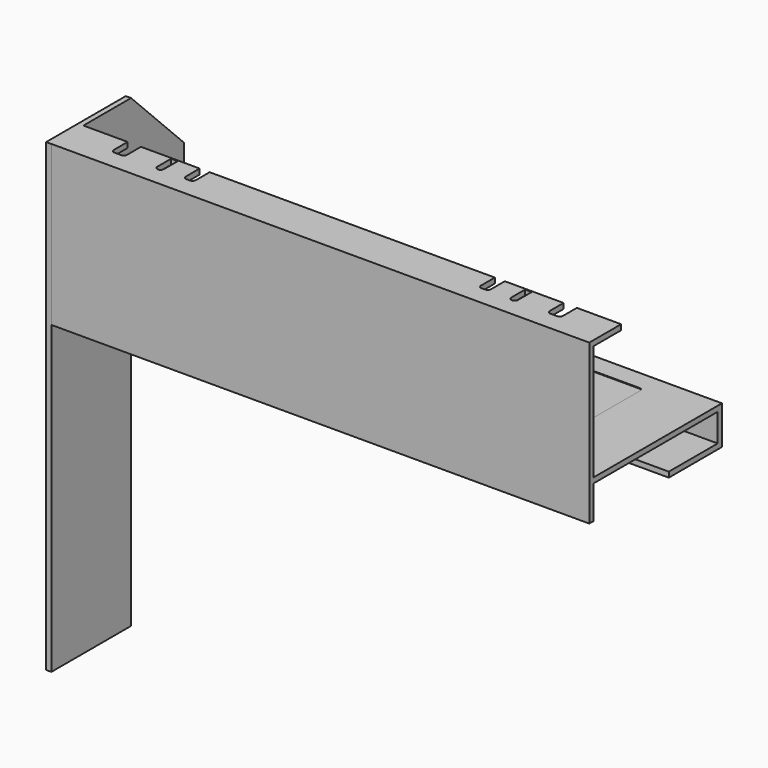
from build123d import *

# Parameters (mm, degrees)
F1_DEPTH = 16
F3_W     = 1620
F3_H     = 484
F4_DEPTH = 16
F5_DEPTH = 14
F6_W     = 184
F6_H     = 16
F6_W_2   = 16
F6_H_2   = 464
F7_DEPTH = 1620
F9_DEPTH = 25


# Not quite as in the source:
# - a feature names something its author has since deleted; it is built from what else it names


with BuildPart() as f1:
    # F0 (on Right) → F1 (new body)
    with BuildSketch(Plane.YZ):
        Polygon((0, 480), (-300, 480), (-300, -920), (0, -920), (0, 0), (200, 0), (200, 280), align=None)
    extrude(amount=-F1_DEPTH)

    # F3 (on offset) → F4 (join)
    with BuildSketch(Plane.XY.offset(100)):
        with Locations((810, -42)):
            Rectangle(F3_W, F3_H)
        with BuildLine():
            Line((200, 140), (680, 140))
            ThreePointArc((680, 140), (687.0710678119, 137.0710678119), (690, 130))
            Line((690, 130), (690, -150))
            ThreePointArc((690, -150), (687.0710678119, -157.0710678119), (680, -160))
            Line((680, -160), (200, -160))
            ThreePointArc((200, -160), (192.9289321881, -157.0710678119), (190, -150))
            Line((190, -150), (190, 130))
            ThreePointArc((190, 130), (192.9289321881, 137.0710678119), (200, 140))
        make_face(mode=Mode.SUBTRACT)
        with BuildLine():
            Line((940, 140), (1420, 140))
            ThreePointArc((1420, 140), (1427.0710678119, 137.0710678119), (1430, 130))
            Line((1430, 130), (1430, -150))
            ThreePointArc((1430, -150), (1427.0710678119, -157.0710678119), (1420, -160))
            Line((1420, -160), (940, -160))
            ThreePointArc((940, -160), (932.9289321881, -157.0710678119), (930, -150))
            Line((930, -150), (930, 130))
            ThreePointArc((930, 130), (932.9289321881, 137.0710678119), (940, 140))
        make_face(mode=Mode.SUBTRACT)
    extrude(amount=F4_DEPTH)

    # F3 (on offset) → F5 (join)
    with BuildSketch(Plane.XY.offset(100)):
        with BuildLine():
            ThreePointArc((690, 130), (687.0710678119, 137.0710678119), (680, 140))
            Line((680, 140), (200, 140))
            ThreePointArc((200, 140), (192.9289321881, 137.0710678119), (190, 130))
            Line((190, 130), (190, -150))
            ThreePointArc((190, -150), (192.9289321881, -157.0710678119), (200, -160))
            Line((200, -160), (680, -160))
            ThreePointArc((680, -160), (687.0710678119, -157.0710678119), (690, -150))
            Line((690, -150), (690, 130))
        make_face()
        with BuildLine():
            ThreePointArc((682, -150), (681.4142135624, -151.4142135624), (680, -152))
            Line((680, -152), (200, -152))
            ThreePointArc((200, -152), (198.5857864376, -151.4142135624), (198, -150))
            Line((198, -150), (198, 130))
            ThreePointArc((198, 130), (198.5857864376, 131.4142135624), (200, 132))
            Line((200, 132), (680, 132))
            ThreePointArc((680, 132), (681.4142135624, 131.4142135624), (682, 130))
            Line((682, 130), (682, -150))
        make_face(mode=Mode.SUBTRACT)
        with BuildLine():
            ThreePointArc((1430, 130), (1427.0710678119, 137.0710678119), (1420, 140))
            Line((1420, 140), (940, 140))
            ThreePointArc((940, 140), (932.9289321881, 137.0710678119), (930, 130))
            Line((930, 130), (930, -150))
            ThreePointArc((930, -150), (932.9289321881, -157.0710678119), (940, -160))
            Line((940, -160), (1420, -160))
            ThreePointArc((1420, -160), (1427.0710678119, -157.0710678119), (1430, -150))
            Line((1430, -150), (1430, 130))
        make_face()
    extrude(amount=F5_DEPTH)

    # F6 (on face) → F7 (join)
    with BuildSketch(Plane.YZ):
        with Locations((92, 8)):
            Rectangle(F6_W, F6_H)
        Polygon((184, 100), (184, 16), (184, 0), (200, 0), (200, 100), align=None)
        with Locations((-291.5103597641, 232)):
            Rectangle(F6_W_2, F6_H_2)
        Polygon((-299.5103597641, 480), (-299.5103597641, 464), (-283.5103597641, 464), (-179.5103597641, 464), (-179.5103597641, 480), align=None)
    extrude(amount=F7_DEPTH)

    # F8 (on face) → F9 (cut)
    with BuildSketch(Plane.XY.offset(480)):
        with BuildLine():
            Line((286.6890323162, -182.5759112835), (266.6890323162, -182.5759112835))
            Line((266.6890323162, -182.5759112835), (266.6890323162, -234.4558739662))
            ThreePointArc((266.6890323162, -234.4558739662), (269.6179645043, -241.5269417781), (276.6890323162, -244.4558739662))
            ThreePointArc((276.6890323162, -244.4558739662), (283.7601001281, -241.5269417781), (286.6890323162, -234.4558739662))
            Line((286.6890323162, -234.4558739662), (286.6890323162, -182.5759112835))
        make_face()
        with BuildLine():
            Line((360.3975868225, -241.5777295828), (370.3975868225, -241.5777295828))
            ThreePointArc((370.3975868225, -241.5777295828), (377.4686546344, -238.6487973947), (380.3975868225, -231.5777295828))
            Line((380.3975868225, -231.5777295828), (380.3975868225, -171.0633635521))
            Line((380.3975868225, -171.0633635521), (350.3975868225, -171.0633635521))
            Line((350.3975868225, -171.0633635521), (350.3975868225, -231.5777295828))
            ThreePointArc((350.3975868225, -231.5777295828), (353.3265190106, -238.6487973947), (360.3975868225, -241.5777295828))
        make_face()
        with BuildLine():
            Line((173.3647221327, -231.5777295828), (173.3647221327, -174.4069010019))
            Line((173.3647221327, -174.4069010019), (133.3647221327, -174.4069010019))
            Line((133.3647221327, -174.4069010019), (133.3647221327, -231.5777295828))
            ThreePointArc((133.3647221327, -231.5777295828), (136.2936543208, -238.6487973947), (143.3647221327, -241.5777295828))
            Line((143.3647221327, -241.5777295828), (163.3647221327, -241.5777295828))
            ThreePointArc((163.3647221327, -241.5777295828), (170.4357899445, -238.6487973947), (173.3647221327, -231.5777295828))
        make_face()
        with BuildLine():
            ThreePointArc((1239.6024131775, -231.5777295828), (1242.5313453656, -238.6487973947), (1249.6024131775, -241.5777295828))
            Line((1249.6024131775, -241.5777295828), (1259.6024131775, -241.5777295828))
            ThreePointArc((1259.6024131775, -241.5777295828), (1266.6734809894, -238.6487973947), (1269.6024131775, -231.5777295828))
            Line((1269.6024131775, -231.5777295828), (1269.6024131775, -171.0633635521))
            Line((1269.6024131775, -171.0633635521), (1239.6024131775, -171.0633635521))
            Line((1239.6024131775, -171.0633635521), (1239.6024131775, -231.5777295828))
        make_face()
        with BuildLine():
            ThreePointArc((1343.3109676838, -244.4558739662), (1350.3820354957, -241.5269417781), (1353.3109676838, -234.4558739662))
            Line((1353.3109676838, -234.4558739662), (1353.3109676838, -182.5759112835))
            Line((1353.3109676838, -182.5759112835), (1333.3109676838, -182.5759112835))
            Line((1333.3109676838, -182.5759112835), (1333.3109676838, -234.4558739662))
            ThreePointArc((1333.3109676838, -234.4558739662), (1336.2398998719, -241.5269417781), (1343.3109676838, -244.4558739662))
        make_face()
        with BuildLine():
            ThreePointArc((1446.6352778673, -231.5777295828), (1449.5642100555, -238.6487973947), (1456.6352778673, -241.5777295828))
            Line((1456.6352778673, -241.5777295828), (1476.6352778673, -241.5777295828))
            ThreePointArc((1476.6352778673, -241.5777295828), (1483.7063456792, -238.6487973947), (1486.6352778673, -231.5777295828))
            Line((1486.6352778673, -231.5777295828), (1486.6352778673, -174.4069010019))
            Line((1486.6352778673, -174.4069010019), (1446.6352778673, -174.4069010019))
            Line((1446.6352778673, -174.4069010019), (1446.6352778673, -231.5777295828))
        make_face()
    extrude(amount=-F9_DEPTH, mode=Mode.SUBTRACT)


solid = f1.part
